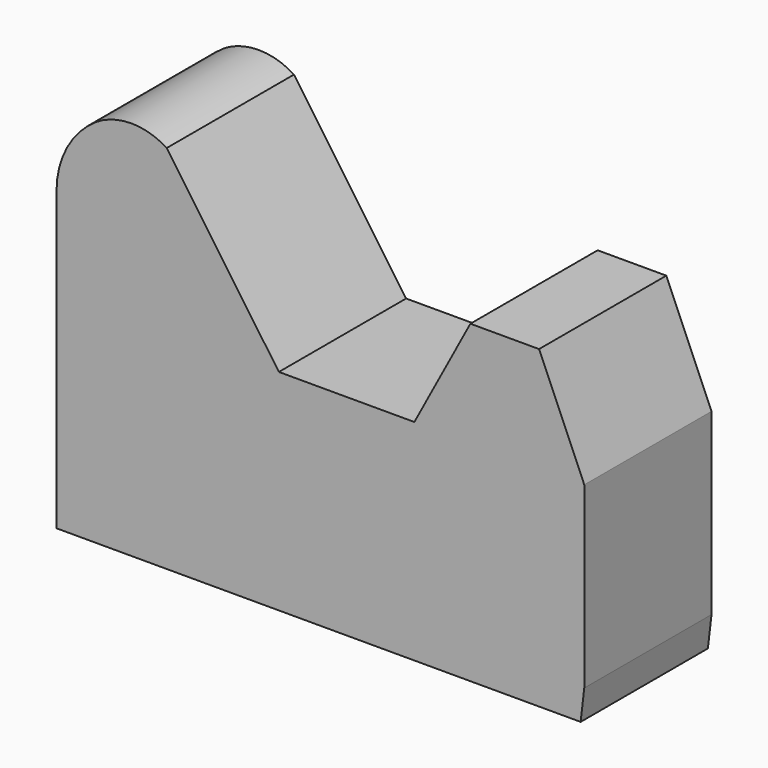
from build123d import *

# Parameters (mm, degrees)
F1_DEPTH = 19.304


# Not quite as in the source:
# - the program builds the solid bodies; features that only make, move or delete a surface that nothing else refers to are left out


with BuildPart() as f1:
    # F0 (on Front) → F1 (new body)
    with BuildSketch(Plane.XZ):
        with BuildLine():
            Line((-26.9875, 34.112624824), (-26.9875, 1.898483652))
            Line((-26.9875, 1.898483652), (26.9875, 1.898483652))
            Line((26.9875, 1.898483652), (37.0624177158, 1.8666714896))
            Line((37.0624177158, 1.8666714896), (37.0624177158, 23.583335802))
            Line((37.0624177158, 23.583335802), (31.5784178674, 36.2954275192))
            Line((31.5784178674, 36.2954275192), (23.2427231967, 36.2954275192))
            Line((23.2427231967, 36.2954275192), (16.4425540715, 23.583335802))
            Line((16.4425540715, 23.583335802), (0, 23.583335802))
            Line((0, 23.583335802), (-13.6097995564, 43.0830909645))
            ThreePointArc((-13.6097995564, 43.0830909645), (-17.8935738167, 44.3218275192), (-22.177348077, 43.0830909645))
            ThreePointArc((-22.177348077, 43.0830909645), (-25.7090842299, 39.2019966984), (-26.9875, 34.112624824))
        make_face()
        Polygon((26.9875, 1.898483652), (-26.9875, 1.898483652), (-26.9875, -1.898483652), (26.9875, -1.898483652), (36.6236940026, -1.898483652), (37.0624177158, 1.8666714896), align=None)
    extrude(amount=F1_DEPTH)


solid = f1.part
